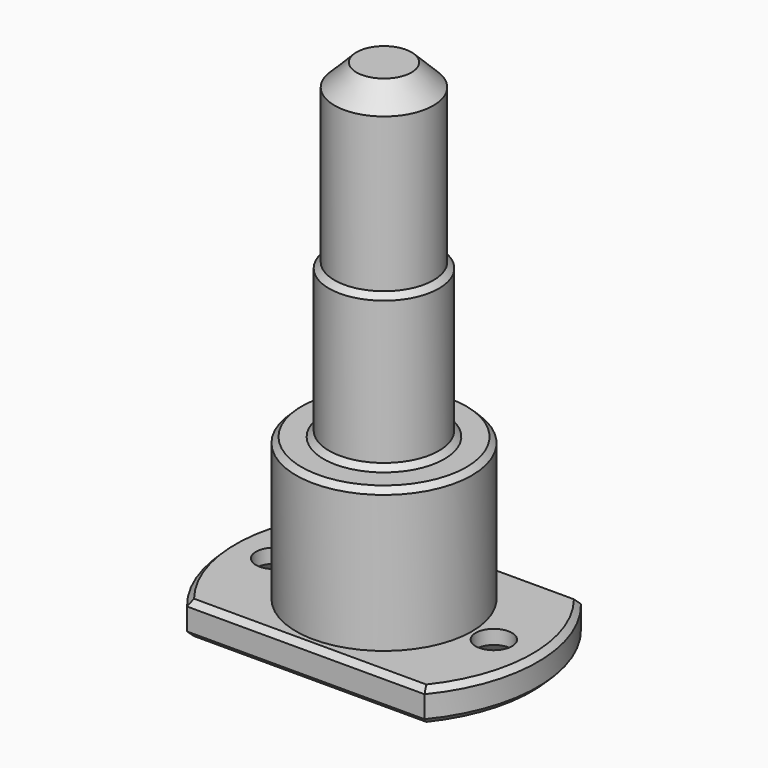
from build123d import *

# Parameters (mm, degrees)
F1_DEPTH       = 3
F3_D           = 3.3
F3_CSINK_D     = 6.72
F3_CSINK_ANGLE = 90
F4_R           = 8
F5_DEPTH       = 13
F6_SIZE2       = 0.5
F6_SIZE        = 0.5
F7_R           = 5
F8_DEPTH       = 14
F9_R           = 4.5
F10_DEPTH      = 16
F11_SIZE2      = 0.49999
F11_SIZE       = 0.49999
F12_SIZE2      = 2
F12_SIZE       = 2


# Not quite as in the source:
# - a fillet or chamfer is up to 0.001 mm smaller than in the source, because OpenCascade refuses the exact size


with BuildPart() as f1:
    # F0 (on Top) → F1 (new body)
    with BuildSketch(Plane.XY):
        with BuildLine():
            Line((10.8069422132, 8.9), (-10.8069422132, 8.9))
            ThreePointArc((-10.8069422132, 8.9), (-14, 0), (-10.8069422132, -8.9))
            Line((-10.8069422132, -8.9), (10.8069422132, -8.9))
            ThreePointArc((10.8069422132, -8.9), (14, 0), (10.8069422132, 8.9))
        make_face()
    extrude(amount=F1_DEPTH)

    # F3 (through all)
    with Locations(Plane(origin=(0, 0, 0), x_dir=(1, 0, 0), z_dir=(0, 0, -1))):
        with Locations((-10, 0), (10, 0)):
            CounterSinkHole(F3_D / 2, F3_CSINK_D / 2, counter_sink_angle=F3_CSINK_ANGLE)

    # F4 (on face) → F5 (join)
    with BuildSketch(Plane.XY.offset(3)):
        Circle(F4_R)
    extrude(amount=F5_DEPTH)

    # F6
    f6_edges = [f1.edges().sort_by_distance(p)[0] for p in [
        (0, 8.9, 3),
        (14, 0, 3),
        (0, -8.9, 3),
        (-14, 0, 3),
    ]]
    chamfer(f6_edges, length=F6_SIZE, length2=F6_SIZE2)

    # F7 (on face) → F8 (join)
    with BuildSketch(Plane.XY.offset(16)):
        Circle(F7_R)
    extrude(amount=F8_DEPTH)

    # F9 (on face) → F10 (join)
    with BuildSketch(Plane.XY.offset(30)):
        Circle(F9_R)
    extrude(amount=F10_DEPTH)

    # F11 (size 0.5 and 0.5 in the source; OpenCascade refuses exactly that, so slightly less here)
    f11_edges = [f1.edges().sort_by_distance(p)[0] for p in [
        (-5, 0, 30),
        (-8, 0, 16),
        (-5, 0, 16),
        (0, 8.9, 0),
        (14, 0, 0),
        (-14, 0, 0),
        (0, -8.9, 0),
    ]]
    chamfer(f11_edges, length=F11_SIZE, length2=F11_SIZE2)

    # F12
    f12_edges = [f1.edges().sort_by_distance(p)[0] for p in [
        (-4.5, 0, 46),
    ]]
    chamfer(f12_edges, length=F12_SIZE, length2=F12_SIZE2)


solid = f1.part
